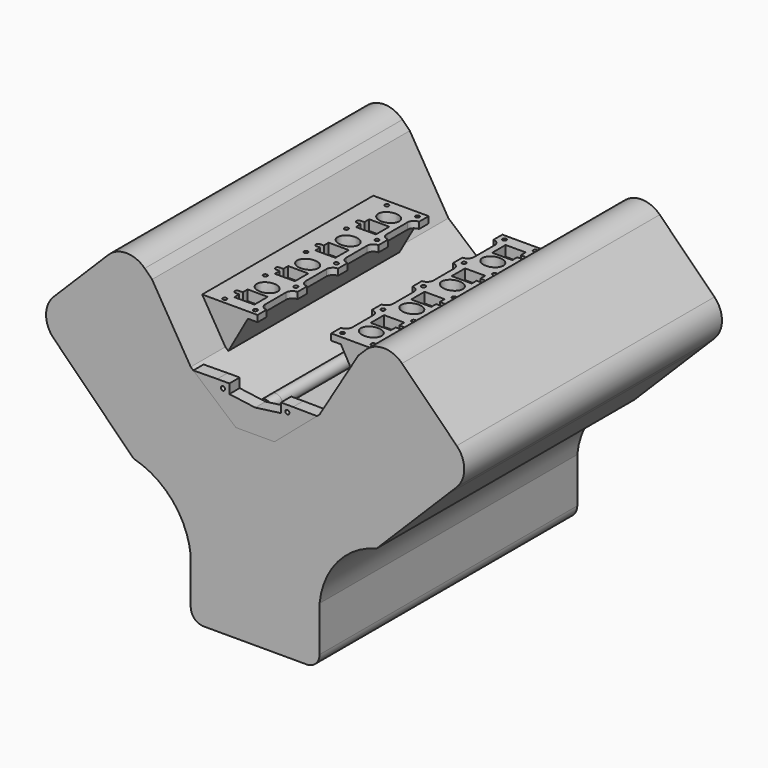
from build123d import *

# Parameters (mm, degrees)
F1_DEPTH  = 635
F2_R      = 4
F3_DEPTH  = 25.4
F6_R      = 12.7
F7_DEPTH  = 25.4
F8_DEPTH  = 584.2
F9_DEPTH  = 558.8
F11_DEPTH = 20.32
F12_W     = 203.2
F12_H     = 105.1513780012
F13_DEPTH = 152.4
F14_R     = 4.0005
F15_DEPTH = 25.4


with BuildPart() as f1:
    # F0 (on Front) → F1 (new body)
    with BuildSketch(Plane.XZ):
        with BuildLine():
            ThreePointArc((-239.7926519853, 132.0295785325), (-162.6701774075, 83.7211039448), (-127, 0))
            Line((-127, 0), (-127, -76.2))
            Line((-127, -76.2), (-127, -88.9))
            ThreePointArc((-127, -88.9), (-119.5605122421, -106.8605122421), (-101.6, -114.3))
            Line((-101.6, -114.3), (101.6, -114.3))
            ThreePointArc((101.6, -114.3), (119.5605122421, -106.8605122421), (127, -88.9))
            Line((127, -88.9), (127, -76.2))
            Line((127, -76.2), (127, 0))
            ThreePointArc((127, 0), (162.6701774075, 83.7211039448), (239.7926519853, 132.0295785325))
            Line((239.7926519853, 132.0295785325), (377.1707570849, 269.4076836321))
            Line((377.1707570849, 269.4076836321), (397.3372515057, 289.5741780528))
            ThreePointArc((397.3372515057, 289.5741780528), (412.2162270214, 325.4952025371), (397.3372515057, 361.4162270214))
            Line((397.3372515057, 361.4162270214), (289.5741780528, 469.1793004742))
            ThreePointArc((289.5741780528, 469.1793004742), (253.6531535686, 484.0582759899), (217.7321290843, 469.1793004742))
            Line((217.7321290843, 469.1793004742), (203.2, 454.6471713899))
            Line((203.2, 454.6471713899), (127, 327.6471713899))
            Line((127, 327.6471713899), (38.1, 251.4471713899))
            Line((38.1, 251.4471713899), (0, 251.4471713899))
            Line((0, 251.4471713899), (-38.1, 251.4471713899))
            Line((-38.1, 251.4471713899), (-127, 327.6471713899))
            Line((-127, 327.6471713899), (-203.2, 454.6471713899))
            Line((-203.2, 454.6471713899), (-217.7321290843, 469.1793004742))
            ThreePointArc((-217.7321290843, 469.1793004742), (-253.6531535686, 484.0582759899), (-289.5741780528, 469.1793004742))
            Line((-289.5741780528, 469.1793004742), (-397.3372515057, 361.4162270214))
            ThreePointArc((-397.3372515057, 361.4162270214), (-412.2162270214, 325.4952025371), (-397.3372515057, 289.5741780528))
            Line((-397.3372515057, 289.5741780528), (-377.1707570849, 269.4076836321))
            Line((-377.1707570849, 269.4076836321), (-239.7926519853, 132.0295785325))
        make_face()
    extrude(amount=F1_DEPTH)


with BuildPart() as f3:
    # F2 (on face) → F3 (new body)
    with BuildSketch(Plane.XZ.offset(635)):
        Polygon((-74.7128501534, 323.7851973335), (-121.92, 323.2928856757), (-38.1, 251.4471713899), (0, 251.4471713899), (38.1, 251.4471713899), (121.92, 323.2928856757), (74.7128501534, 323.7851973335), (50.8, 323.7851973335), (50.8, 305.3245832334), (0, 298.4288622747), (-50.8, 305.3245832334), (-50.8, 323.7851973335), align=None)
        with Locations((-63.5, 311.0851973335)):
            Circle(F2_R, mode=Mode.SUBTRACT)
        with Locations((63.5, 311.0851973335)):
            Circle(F2_R, mode=Mode.SUBTRACT)
    extrude(amount=-F3_DEPTH)

    # F6 (on offset) → F7 (join)
    with BuildSketch(Plane.XZ.offset(584.2)):
        with Locations((0, 289.5471713899)):
            Circle(F6_R)
    extrude(amount=F7_DEPTH)

    # F6 (on offset) → F8 (join, through all)
    with BuildSketch(Plane.XZ.offset(584.2)):
        with Locations((0, 289.5471713899)):
            Circle(F6_R)
    extrude(amount=-F8_DEPTH)


with BuildPart() as f9:
    # F5 (on offset) → F9 (new body)
    with BuildSketch(Plane.XZ.offset(584.2)):
        Polygon((-63.5, 403.8471713899), (-190.5, 403.8471713899), (-190.5, 298.4539927969), (-134.6899344925, 298.4539927969), (-82.55, 391.1471713899), (-63.5, 391.1471713899), align=None)
    extrude(amount=-F9_DEPTH)


with BuildPart() as f9b:
    # F5 (on offset) → F9, piece 2 (new body)
    with BuildSketch(Plane.XZ.offset(584.2)):
        Polygon((63.5, 391.1471713899), (82.55, 391.1471713899), (134.6899344925, 298.4539927969), (190.5, 298.4539927969), (190.5, 403.8471713899), (63.5, 403.8471713899), align=None)
    extrude(amount=-F9_DEPTH)


with BuildPart() as f11_tool:
    # F10 (on face) → F11 (new body)
    with BuildSketch(Plane.XY.offset(403.8471713899)):
        with BuildLine():
            Line((-128.524, -226.3093780012), (-88.9, -226.3093780012))
            Line((-88.9, -226.3093780012), (-88.9, -193.2893780012))
            Line((-88.9, -193.2893780012), (-128.524, -193.2893780012))
            Line((-128.524, -193.2893780012), (-128.524, -205.3543780012))
            Line((-128.524, -205.3543780012), (-136.017, -205.3543780012))
            ThreePointArc((-136.017, -205.3543780012), (-140.462, -209.7993780012), (-136.017, -214.2443780012))
            Line((-136.017, -214.2443780012), (-128.524, -214.2443780012))
            Line((-128.524, -214.2443780012), (-128.524, -226.3093780012))
        make_face()
        with BuildLine():
            Line((-50.685784769, -151.8238780012), (-63.5, -151.8238780012))
            ThreePointArc((-63.5, -151.8238780012), (-72.4802561211, -155.5436218801), (-76.2, -164.5238780012))
            Line((-76.2, -164.5238780012), (-76.2, -215.3238780012))
            ThreePointArc((-76.2, -215.3238780012), (-72.4802561211, -224.3041341222), (-63.5, -228.0238780012))
            Line((-63.5, -228.0238780012), (-50.685784769, -228.0238780012))
            Line((-50.685784769, -228.0238780012), (-50.685784769, -151.8238780012))
        make_face()
        with BuildLine():
            add(Edge.make_bspline(
                [(-88.011, -170.0483780012), (-88.011, -140.7923078105), (-119.0625, -155.4203429059), (-150.114, -170.0483780012), (-119.0625, -184.6764130965), (-88.011, -199.3044481918), (-88.011, -170.0483780012)],
                knots=[0, 0, 0, 2.0943951024, 2.0943951024, 4.1887902048, 4.1887902048, 6.2831853072, 6.2831853072, 6.2831853072], degree=2, weights=[1, 0.5, 1, 0.5, 1, 0.5, 1]))
        make_face()
        with BuildLine():
            ThreePointArc((-76.2, -315.1458780012), (-72.4802561211, -324.1261341222), (-63.5, -327.8458780012))
            Line((-63.5, -327.8458780012), (-50.685784769, -327.8458780012))
            Line((-50.685784769, -327.8458780012), (-50.685784769, -251.6458780012))
            Line((-50.685784769, -251.6458780012), (-63.5, -251.6458780012))
            ThreePointArc((-63.5, -251.6458780012), (-72.4802561211, -255.3656218801), (-76.2, -264.3458780012))
            Line((-76.2, -264.3458780012), (-76.2, -315.1458780012))
        make_face()
        with BuildLine():
            Line((-128.524, -293.1113780012), (-128.524, -305.1763780012))
            Line((-128.524, -305.1763780012), (-136.017, -305.1763780012))
            ThreePointArc((-136.017, -305.1763780012), (-140.462, -309.6213780012), (-136.017, -314.0663780012))
            Line((-136.017, -314.0663780012), (-128.524, -314.0663780012))
            Line((-128.524, -314.0663780012), (-128.524, -326.1313780012))
            Line((-128.524, -326.1313780012), (-88.9, -326.1313780012))
            Line((-88.9, -326.1313780012), (-88.9, -293.1113780012))
            Line((-88.9, -293.1113780012), (-128.524, -293.1113780012))
        make_face()
        with BuildLine():
            add(Edge.make_bspline(
                [(-88.011, -269.8703780012), (-88.011, -240.6143078105), (-119.0625, -255.2423429059), (-150.114, -269.8703780012), (-119.0625, -284.4984130965), (-88.011, -299.1264481918), (-88.011, -269.8703780012)],
                knots=[0, 0, 0, 2.0943951024, 2.0943951024, 4.1887902048, 4.1887902048, 6.2831853072, 6.2831853072, 6.2831853072], degree=2, weights=[1, 0.5, 1, 0.5, 1, 0.5, 1]))
        make_face()
        with BuildLine():
            ThreePointArc((-76.2, -414.9678780012), (-72.4802561211, -423.9481341222), (-63.5, -427.6678780012))
            Line((-63.5, -427.6678780012), (-50.685784769, -427.6678780012))
            Line((-50.685784769, -427.6678780012), (-50.685784769, -351.4678780012))
            Line((-50.685784769, -351.4678780012), (-63.5, -351.4678780012))
            ThreePointArc((-63.5, -351.4678780012), (-72.4802561211, -355.1876218801), (-76.2, -364.1678780012))
            Line((-76.2, -364.1678780012), (-76.2, -414.9678780012))
        make_face()
        with BuildLine():
            Line((-128.524, -392.9333780012), (-128.524, -404.9983780012))
            Line((-128.524, -404.9983780012), (-136.017, -404.9983780012))
            ThreePointArc((-136.017, -404.9983780012), (-140.462, -409.4433780012), (-136.017, -413.8883780012))
            Line((-136.017, -413.8883780012), (-128.524, -413.8883780012))
            Line((-128.524, -413.8883780012), (-128.524, -425.9533780012))
            Line((-128.524, -425.9533780012), (-88.9, -425.9533780012))
            Line((-88.9, -425.9533780012), (-88.9, -392.9333780012))
            Line((-88.9, -392.9333780012), (-128.524, -392.9333780012))
        make_face()
        with BuildLine():
            add(Edge.make_bspline(
                [(-88.011, -369.6923780012), (-88.011, -340.4363078105), (-119.0625, -355.0643429059), (-150.114, -369.6923780012), (-119.0625, -384.3204130965), (-88.011, -398.9484481918), (-88.011, -369.6923780012)],
                knots=[0, 0, 0, 2.0943951024, 2.0943951024, 4.1887902048, 4.1887902048, 6.2831853072, 6.2831853072, 6.2831853072], degree=2, weights=[1, 0.5, 1, 0.5, 1, 0.5, 1]))
        make_face()
        with BuildLine():
            ThreePointArc((-76.2, -514.7898780012), (-72.4802561211, -523.7701341222), (-63.5, -527.4898780012))
            Line((-63.5, -527.4898780012), (-50.685784769, -527.4898780012))
            Line((-50.685784769, -527.4898780012), (-50.685784769, -451.2898780012))
            Line((-50.685784769, -451.2898780012), (-63.5, -451.2898780012))
            ThreePointArc((-63.5, -451.2898780012), (-72.4802561211, -455.0096218801), (-76.2, -463.9898780012))
            Line((-76.2, -463.9898780012), (-76.2, -514.7898780012))
        make_face()
        with BuildLine():
            Line((-128.524, -492.7553780012), (-128.524, -504.8203780012))
            Line((-128.524, -504.8203780012), (-136.017, -504.8203780012))
            ThreePointArc((-136.017, -504.8203780012), (-140.462, -509.2653780012), (-136.017, -513.7103780012))
            Line((-136.017, -513.7103780012), (-128.524, -513.7103780012))
            Line((-128.524, -513.7103780012), (-128.524, -525.7753780012))
            Line((-128.524, -525.7753780012), (-88.9, -525.7753780012))
            Line((-88.9, -525.7753780012), (-88.9, -492.7553780012))
            Line((-88.9, -492.7553780012), (-128.524, -492.7553780012))
        make_face()
        with BuildLine():
            add(Edge.make_bspline(
                [(-88.011, -469.5143780012), (-88.011, -440.2583078105), (-119.0625, -454.8863429059), (-150.114, -469.5143780012), (-119.0625, -484.1424130965), (-88.011, -498.7704481918), (-88.011, -469.5143780012)],
                knots=[0, 0, 0, 2.0943951024, 2.0943951024, 4.1887902048, 4.1887902048, 6.2831853072, 6.2831853072, 6.2831853072], degree=2, weights=[1, 0.5, 1, 0.5, 1, 0.5, 1]))
        make_face()
        with BuildLine():
            Line((128.524, -328.6713780012), (88.9, -328.6713780012))
            Line((88.9, -328.6713780012), (88.9, -361.6913780012))
            Line((88.9, -361.6913780012), (128.524, -361.6913780012))
            Line((128.524, -361.6913780012), (128.524, -349.6263780012))
            Line((128.524, -349.6263780012), (136.017, -349.6263780012))
            ThreePointArc((136.017, -349.6263780012), (140.462, -345.1813780012), (136.017, -340.7363780012))
            Line((136.017, -340.7363780012), (128.524, -340.7363780012))
            Line((128.524, -340.7363780012), (128.524, -328.6713780012))
        make_face()
        with BuildLine():
            Line((76.2, -390.4568780012), (76.2, -339.6568780012))
            ThreePointArc((76.2, -339.6568780012), (72.4802561211, -330.6766218801), (63.5, -326.9568780012))
            Line((63.5, -326.9568780012), (50.685784769, -326.9568780012))
            Line((50.685784769, -326.9568780012), (50.685784769, -403.1568780012))
            Line((50.685784769, -403.1568780012), (63.5, -403.1568780012))
            ThreePointArc((63.5, -403.1568780012), (72.4802561211, -399.4371341222), (76.2, -390.4568780012))
        make_face()
        with BuildLine():
            ThreePointArc((63.5, -203.5128780012), (72.4802561211, -199.7931341222), (76.2, -190.8128780012))
            Line((76.2, -190.8128780012), (76.2, -140.0128780012))
            ThreePointArc((76.2, -140.0128780012), (72.4802561211, -131.0326218801), (63.5, -127.3128780012))
            Line((63.5, -127.3128780012), (50.685784769, -127.3128780012))
            Line((50.685784769, -127.3128780012), (50.685784769, -203.5128780012))
            Line((50.685784769, -203.5128780012), (63.5, -203.5128780012))
        make_face()
        with BuildLine():
            add(Edge.make_bspline(
                [(88.011, -484.7543780012), (88.011, -514.0104481918), (119.0625, -499.3824130965), (150.114, -484.7543780012), (119.0625, -470.1263429059), (88.011, -455.4983078105), (88.011, -484.7543780012)],
                knots=[0, 0, 0, 2.0943951024, 2.0943951024, 4.1887902048, 4.1887902048, 6.2831853072, 6.2831853072, 6.2831853072], degree=2, weights=[1, 0.5, 1, 0.5, 1, 0.5, 1]))
        make_face()
        with BuildLine():
            Line((50.685784769, -227.1348780012), (50.685784769, -303.3348780012))
            Line((50.685784769, -303.3348780012), (63.5, -303.3348780012))
            ThreePointArc((63.5, -303.3348780012), (72.4802561211, -299.6151341222), (76.2, -290.6348780012))
            Line((76.2, -290.6348780012), (76.2, -239.8348780012))
            ThreePointArc((76.2, -239.8348780012), (72.4802561211, -230.8546218801), (63.5, -227.1348780012))
            Line((63.5, -227.1348780012), (50.685784769, -227.1348780012))
        make_face()
        with BuildLine():
            Line((128.524, -428.4933780012), (88.9, -428.4933780012))
            Line((88.9, -428.4933780012), (88.9, -461.5133780012))
            Line((88.9, -461.5133780012), (128.524, -461.5133780012))
            Line((128.524, -461.5133780012), (128.524, -449.4483780012))
            Line((128.524, -449.4483780012), (136.017, -449.4483780012))
            ThreePointArc((136.017, -449.4483780012), (140.462, -445.0033780012), (136.017, -440.5583780012))
            Line((136.017, -440.5583780012), (128.524, -440.5583780012))
            Line((128.524, -440.5583780012), (128.524, -428.4933780012))
        make_face()
        with BuildLine():
            Line((128.524, -228.8493780012), (88.9, -228.8493780012))
            Line((88.9, -228.8493780012), (88.9, -261.8693780012))
            Line((88.9, -261.8693780012), (128.524, -261.8693780012))
            Line((128.524, -261.8693780012), (128.524, -249.8043780012))
            Line((128.524, -249.8043780012), (136.017, -249.8043780012))
            ThreePointArc((136.017, -249.8043780012), (140.462, -245.3593780012), (136.017, -240.9143780012))
            Line((136.017, -240.9143780012), (128.524, -240.9143780012))
            Line((128.524, -240.9143780012), (128.524, -228.8493780012))
        make_face()
        with BuildLine():
            Line((128.524, -129.0273780012), (88.9, -129.0273780012))
            Line((88.9, -129.0273780012), (88.9, -162.0473780012))
            Line((88.9, -162.0473780012), (128.524, -162.0473780012))
            Line((128.524, -162.0473780012), (128.524, -149.9823780012))
            Line((128.524, -149.9823780012), (136.017, -149.9823780012))
            ThreePointArc((136.017, -149.9823780012), (140.462, -145.5373780012), (136.017, -141.0923780012))
            Line((136.017, -141.0923780012), (128.524, -141.0923780012))
            Line((128.524, -141.0923780012), (128.524, -129.0273780012))
        make_face()
        with BuildLine():
            add(Edge.make_bspline(
                [(88.011, -185.2883780012), (88.011, -214.5444481918), (119.0625, -199.9164130965), (150.114, -185.2883780012), (119.0625, -170.6603429059), (88.011, -156.0323078105), (88.011, -185.2883780012)],
                knots=[0, 0, 0, 2.0943951024, 2.0943951024, 4.1887902048, 4.1887902048, 6.2831853072, 6.2831853072, 6.2831853072], degree=2, weights=[1, 0.5, 1, 0.5, 1, 0.5, 1]))
        make_face()
        with BuildLine():
            Line((50.685784769, -426.7788780012), (50.685784769, -502.9788780012))
            Line((50.685784769, -502.9788780012), (63.5, -502.9788780012))
            ThreePointArc((63.5, -502.9788780012), (72.4802561211, -499.2591341222), (76.2, -490.2788780012))
            Line((76.2, -490.2788780012), (76.2, -439.4788780012))
            ThreePointArc((76.2, -439.4788780012), (72.4802561211, -430.4986218801), (63.5, -426.7788780012))
            Line((63.5, -426.7788780012), (50.685784769, -426.7788780012))
        make_face()
        with BuildLine():
            add(Edge.make_bspline(
                [(88.011, -384.9323780012), (88.011, -414.1884481918), (119.0625, -399.5604130965), (150.114, -384.9323780012), (119.0625, -370.3043429059), (88.011, -355.6763078105), (88.011, -384.9323780012)],
                knots=[0, 0, 0, 2.0943951024, 2.0943951024, 4.1887902048, 4.1887902048, 6.2831853072, 6.2831853072, 6.2831853072], degree=2, weights=[1, 0.5, 1, 0.5, 1, 0.5, 1]))
        make_face()
        with BuildLine():
            add(Edge.make_bspline(
                [(88.011, -285.1103780012), (88.011, -314.3664481918), (119.0625, -299.7384130965), (150.114, -285.1103780012), (119.0625, -270.4823429059), (88.011, -255.8543078105), (88.011, -285.1103780012)],
                knots=[0, 0, 0, 2.0943951024, 2.0943951024, 4.1887902048, 4.1887902048, 6.2831853072, 6.2831853072, 6.2831853072], degree=2, weights=[1, 0.5, 1, 0.5, 1, 0.5, 1]))
        make_face()
    extrude(amount=-F11_DEPTH)


with BuildPart() as f9_1:
    add(f9.part)

    # F11: cut by f11_tool
    add(f11_tool.part, mode=Mode.SUBTRACT)


with BuildPart() as f9b_1:
    add(f9b.part)

    # F11: cut by f11_tool
    add(f11_tool.part, mode=Mode.SUBTRACT)


with BuildPart() as f13_tool:
    # F12 (on face) → F13 (new body)
    with BuildSketch(Plane.XY.offset(403.8471713899)):
        Polygon((-203.2, -127.9478780012), (0, -127.9478780012), (0, -105.1513780012), (0, 0), (-203.2, 0), align=None)
        with Locations((101.6, -52.5756890006)):
            Rectangle(F12_W, F12_H)
        Polygon((203.2, -526.8548780012), (0, -526.8548780012), (0, -549.6513780012), (0, -584.2), (0, -653.0923843384), (203.2, -653.0923843384), align=None)
        Polygon((0, -584.2), (0, -549.6513780012), (-203.2, -549.6513780012), (-203.2, -653.0923843384), (0, -653.0923843384), align=None)
    extrude(amount=-F13_DEPTH)


with BuildPart() as f9_2:
    add(f9_1.part)

    # F13: cut by f13_tool
    add(f13_tool.part, mode=Mode.SUBTRACT)


with BuildPart() as f9b_2:
    add(f9b_1.part)

    # F13: cut by f13_tool
    add(f13_tool.part, mode=Mode.SUBTRACT)


with BuildPart() as f15_tool:
    # F14 (on face) → F15 (new body)
    with BuildSketch(Plane.XY.offset(403.8471713899)):
        with Locations((-76.2, -539.1103780012)):
            Circle(F14_R)
        with Locations((-76.2, -439.2883780012)):
            Circle(F14_R)
        with Locations((-76.2, -339.4663780012)):
            Circle(F14_R)
        with Locations((-76.2, -239.6443780012)):
            Circle(F14_R)
        with Locations((-76.2, -139.8223780012)):
            Circle(F14_R)
        with Locations((-136.525, -539.1103780012)):
            Circle(F14_R)
        with Locations((-136.525, -439.2883780012)):
            Circle(F14_R)
        with Locations((-136.525, -339.4663780012)):
            Circle(F14_R)
        with Locations((-136.525, -239.6443780012)):
            Circle(F14_R)
        with Locations((-136.525, -139.8223780012)):
            Circle(F14_R)
        with Locations((76.2, -115.6923780012)):
            Circle(F14_R)
        with Locations((76.2, -215.5143780012)):
            Circle(F14_R)
        with Locations((76.2, -315.3363780012)):
            Circle(F14_R)
        with Locations((76.2, -415.1583780012)):
            Circle(F14_R)
        with Locations((76.2, -514.9803780012)):
            Circle(F14_R)
        with Locations((136.525, -115.6923780012)):
            Circle(F14_R)
        with Locations((136.525, -215.5143780012)):
            Circle(F14_R)
        with Locations((136.525, -315.3363780012)):
            Circle(F14_R)
        with Locations((136.525, -415.1583780012)):
            Circle(F14_R)
        with Locations((136.525, -514.9803780012)):
            Circle(F14_R)
    extrude(amount=-F15_DEPTH)


with BuildPart() as f9_3:
    add(f9_2.part)

    # F15: cut by f15_tool
    add(f15_tool.part, mode=Mode.SUBTRACT)


with BuildPart() as f9b_3:
    add(f9b_2.part)

    # F15: cut by f15_tool
    add(f15_tool.part, mode=Mode.SUBTRACT)


solid = Compound([f1.part, f3.part, f9_3.part, f9b_3.part])
